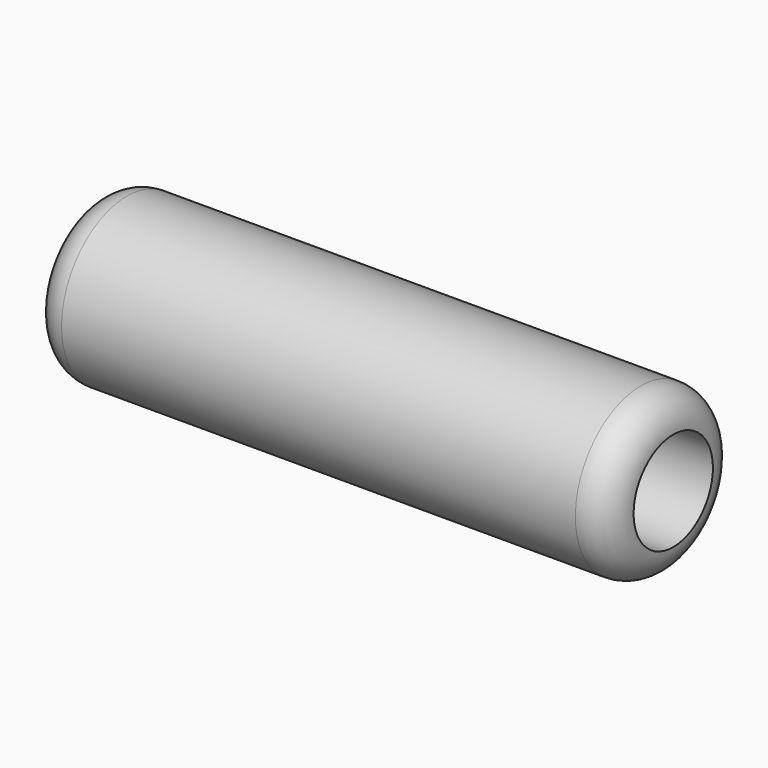
from build123d import *

# Parameters (mm, degrees)
F3_R = 6.34999
F4_R = 6.35


# Not quite as in the source:
# - a fillet or chamfer is up to 0.001 mm smaller than in the source, because OpenCascade refuses the exact size


with BuildPart() as f2:
    # F0 (on Front) → F2 (revolve)
    with BuildSketch(Plane.XZ):
        Polygon((69.7922009419, 11.5239060186), (-39.7579990581, 11.5239060186), (-39.7579990581, 18.8685089484), (-43.7203990581, 18.8685089484), (-43.7203990581, 5.1739060186), (69.7922009419, 5.1739060186), align=None)
    revolve(axis=Axis((18.9415253699, 0, 21.2497589484), (1, 0, 0)))

    # F3 (radius 6.35 in the source; OpenCascade refuses exactly that, so slightly less here)
    f3_edges = [f2.edges().sort_by_distance(p)[0] for p in [
        (69.792201, 0, 37.325612),
    ]]
    fillet(f3_edges, radius=F3_R)

    # F4
    f4_edges = [f2.edges().sort_by_distance(p)[0] for p in [
        (-43.720399, 0, 37.325612),
    ]]
    fillet(f4_edges, radius=F4_R)


solid = f2.part
